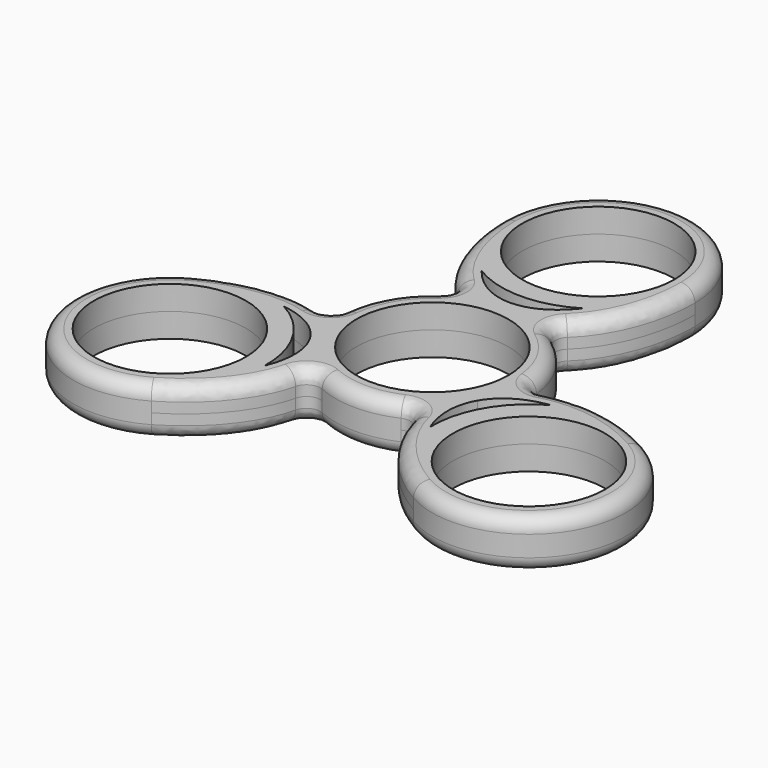
from build123d import *

# Parameters (mm, degrees)
F0_R     = 11
F1_DEPTH = 3.5
F2_F1_R  = 2
F2_F2_R  = 2


with BuildPart() as f1:
    # F0 (on Top) → F1 (new body, symmetric)
    with BuildSketch(Plane.XY):
        with BuildLine():
            add(Edge.make_bspline(
                [(-14, 30), (-14, 17.8068938204), (-5.8323690663, 12.7272727273)],
                knots=[1.5707963268, 1.5707963268, 1.5707963268, 2.7118929874, 2.7118929874, 2.7118929874], degree=2, weights=[1, 0.841604952, 1]))
            ThreePointArc((-5.8323690663, 12.7272727273), (-12.124355653, 7), (-13.9383260359, -1.312656588))
            ThreePointArc((-13.9383260359, -1.312656588), (-13.9167685556, -1.5243204946), (-13.8919969881, -1.7356323585))
            ThreePointArc((-13.8919969881, -1.7356323585), (-13.2718138334, -4.4563390324), (-12.1243556028, -7.0000000869))
            ThreePointArc((-12.1243556028, -7.0000000869), (-10.4952096602, -9.265558493), (-8.4491002081, -11.1630061217))
            ThreePointArc((-8.4491002081, -11.1630061217), (-8.2784845497, -11.2901148604), (-8.1059569696, -11.4146161393))
            ThreePointArc((-8.1059569696, -11.4146161393), (0, -14), (8.1059569696, -11.4146161393))
            ThreePointArc((8.1059569696, -11.4146161393), (8.2784845497, -11.2901148604), (8.4491002081, -11.1630061217))
            ThreePointArc((8.4491002081, -11.1630061217), (10.4952095782, -9.2655585859), (12.1243554789, -7.0000003015))
            ThreePointArc((12.1243554789, -7.0000003015), (13.271813794, -4.4563391499), (13.8919969881, -1.7356323585))
            ThreePointArc((13.8919969881, -1.7356323585), (13.9167685556, -1.5243204946), (13.9383260359, -1.312656588))
            ThreePointArc((13.9383260359, -1.312656588), (12.124355653, 7), (5.8323690663, 12.7272727273))
            add(Edge.make_bspline(
                [(5.8323690663, 12.7272727273), (14, 17.8068938204), (14, 30)],
                knots=[3.5712923197, 3.5712923197, 3.5712923197, 4.7123889804, 4.7123889804, 4.7123889804], degree=2, weights=[1, 0.841604952, 1]))
            ThreePointArc((14, 30), (0, 44), (-14, 30))
        make_face()
        Circle(F0_R, mode=Mode.SUBTRACT)
        with BuildLine():
            add(Edge.make_bspline(
                [(-7.3333333333, 18.07430412), (0, 8.533747416), (7.3333333333, 18.07430412)],
                knots=[2.4118649974, 2.4118649974, 2.4118649974, 3.8713203098, 3.8713203098, 3.8713203098], degree=2, weights=[1, 0.7453559925, 1]))
            ThreePointArc((-7.3333333333, 18.07430412), (0, 16), (7.3333333333, 18.07430412))
        make_face(mode=Mode.SUBTRACT)
        with Locations((0, 30)):
            Circle(F0_R, mode=Mode.SUBTRACT)
        with BuildLine():
            ThreePointArc((-13.8919969881, -1.7356323585), (-13.9167685556, -1.5243204946), (-13.9383260359, -1.312656588))
            add(Edge.make_bspline(
                [(-13.9383260359, -1.312656588), (-22.421222411, 3.2209087428), (-32.9807621135, -2.875644347)],
                knots=[3.5712923197, 3.5712923197, 3.5712923197, 4.7123889804, 4.7123889804, 4.7123889804], degree=2, weights=[1, 0.841604952, 1]))
            ThreePointArc((-32.9807621135, -2.875644347), (-38.1051177665, -22), (-18.9807621135, -27.124355653))
            add(Edge.make_bspline(
                [(-18.9807621135, -27.124355653), (-8.421222411, -21.0278025632), (-8.1059569696, -11.4146161393)],
                knots=[1.5707963268, 1.5707963268, 1.5707963268, 2.7118929874, 2.7118929874, 2.7118929874], degree=2, weights=[1, 0.841604952, 1]))
            ThreePointArc((-8.1059569696, -11.4146161393), (-8.2784845497, -11.2901148604), (-8.4491002081, -11.1630061217))
            ThreePointArc((-8.4491002081, -11.1630061217), (-10.4952096602, -9.265558493), (-12.1243556028, -7.0000000869))
            ThreePointArc((-12.1243556028, -7.0000000869), (-13.2718138334, -4.4563390324), (-13.8919969881, -1.7356323585))
        make_face()
        with Locations((-25.9807621135, -15)):
            Circle(F0_R, mode=Mode.SUBTRACT)
        with BuildLine():
            add(Edge.make_bspline(
                [(-12.1243556028, -7.0000000869), (-14.2251686452, -3.3612850489), (-19.3194731903, -2.6862990989)],
                knots=[3.1415926445, 3.1415926445, 3.1415926445, 3.8713203098, 3.8713203098, 3.8713203098], degree=2, weights=[1, 0.9341723573, 1]))
            add(Edge.make_bspline(
                [(-11.986139857, -15.3880050211), (-10.0235426179, -10.6387150253), (-12.1243556028, -7.0000000869)],
                knots=[2.4118649974, 2.4118649974, 2.4118649974, 3.1415926445, 3.1415926445, 3.1415926445], degree=2, weights=[1, 0.9341723606, 1]))
            ThreePointArc((-11.986139857, -15.3880050211), (-13.8564064606, -8), (-19.3194731903, -2.6862990989))
        make_face(mode=Mode.SUBTRACT)
        with BuildLine():
            add(Edge.make_bspline(
                [(32.9807621135, -2.875644347), (22.421222411, 3.2209087428), (13.9383260359, -1.312656588)],
                knots=[1.5707963268, 1.5707963268, 1.5707963268, 2.7118929874, 2.7118929874, 2.7118929874], degree=2, weights=[1, 0.841604952, 1]))
            ThreePointArc((13.9383260359, -1.312656588), (13.9167685556, -1.5243204946), (13.8919969881, -1.7356323585))
            ThreePointArc((13.8919969881, -1.7356323585), (13.271813794, -4.4563391499), (12.1243554789, -7.0000003015))
            ThreePointArc((12.1243554789, -7.0000003015), (10.4952095782, -9.2655585859), (8.4491002081, -11.1630061217))
            ThreePointArc((8.4491002081, -11.1630061217), (8.2784845497, -11.2901148604), (8.1059569696, -11.4146161393))
            add(Edge.make_bspline(
                [(8.1059569696, -11.4146161393), (8.421222411, -21.0278025632), (18.9807621135, -27.124355653)],
                knots=[3.5712923197, 3.5712923197, 3.5712923197, 4.7123889804, 4.7123889804, 4.7123889804], degree=2, weights=[1, 0.841604952, 1]))
            ThreePointArc((18.9807621135, -27.124355653), (38.1051177665, -22), (32.9807621135, -2.875644347))
        make_face()
        with Locations((25.9807621135, -15)):
            Circle(F0_R, mode=Mode.SUBTRACT)
        with BuildLine():
            add(Edge.make_bspline(
                [(12.1243554789, -7.0000003015), (10.0235426843, -10.6387151858), (11.986139857, -15.3880050211)],
                knots=[3.1415926852, 3.1415926852, 3.1415926852, 3.8713203098, 3.8713203098, 3.8713203098], degree=2, weights=[1, 0.9341723646, 1]))
            add(Edge.make_bspline(
                [(19.3194731903, -2.6862990989), (14.225168473, -3.3612850717), (12.1243554789, -7.0000003015)],
                knots=[2.4118649974, 2.4118649974, 2.4118649974, 3.1415926852, 3.1415926852, 3.1415926852], degree=2, weights=[1, 0.9341723533, 1]))
            ThreePointArc((19.3194731903, -2.6862990989), (13.8564064606, -8), (11.986139857, -15.3880050211))
        make_face(mode=Mode.SUBTRACT)
    extrude(amount=F1_DEPTH, both=True)

    # F2: fillet of radius 2 on 40 edges, made by hand

    # F2_f1
    f2_f1_edges = [f1.edges().sort_by_distance(p)[0] for p in [
        (-5.8323690663, 12.7272727273, -1.75),
        (-8.1059569696, -11.4146161393, -1.75),
        (-13.9383260359, -1.312656588, -1.75),
        (-13.9383260359, -1.312656588, 1.75),
        (-5.8323690663, 12.7272727273, 1.75),
        (8.1059569696, -11.4146161393, -1.75),
        (13.9383260359, -1.312656588, -1.75),
        (5.8323690663, 12.7272727273, -1.75),
        (5.8323690663, 12.7272727273, 1.75),
        (13.9383260359, -1.312656588, 1.75),
        (8.1059569696, -11.4146161393, 1.75),
        (-8.1059569696, -11.4146161393, 1.75),
    ]]
    fillet(f2_f1_edges, radius=F2_F1_R)

    # F2_f2
    f2_f2_edges = [f1.edges().sort_by_distance(p)[0] for p in [
        (-12.446293522, 21.3005366984, -3.5),
        (0, 44, -3.5),
        (0, 44, 3.5),
        (-38.1051177665, -22, -3.5),
        (-38.1051177665, -22, 3.5),
        (-12.223659134, -21.4290747222, -3.5),
        (-12.124355653, 7, -3.5),
        (-12.124355653, 7, 3.5),
        (-24.6699526561, 0.1285380239, -3.5),
        (12.223659134, -21.4290747222, -3.5),
        (38.1051177665, -22, -3.5),
        (38.1051177665, -22, 3.5),
        (12.124355653, 7, -3.5),
        (12.124355653, 7, 3.5),
        (12.223659134, -21.4290747222, 3.5),
        (24.6699526561, 0.1285380239, 3.5),
        (24.6699526561, 0.1285380239, -3.5),
        (-24.6699526561, 0.1285380239, 3.5),
        (-12.223659134, -21.4290747222, 3.5),
        (12.446293522, 21.3005366984, 3.5),
        (-12.446293522, 21.3005366984, 3.5),
        (12.446293522, 21.3005366984, -3.5),
        (7.385566687, 12.8300381313, -3.5),
        (-7.3855666873, 12.8300381307, 3.5),
        (7.385566687, 12.8300381313, 3.5),
        (-7.4183556091, -12.8111074378, 3.5),
        (-14.8039222962, -0.018930693, 3.5),
        (14.8039222968, -0.0189306934, -3.5),
        (14.8039222968, -0.0189306934, 3.5),
        (7.4183556097, -12.8111074381, 3.5),
        (7.4183556097, -12.8111074381, -3.5),
        (-14.8039222969, -0.0189306932, -3.5),
        (-7.385566687, 12.8300381313, -3.5),
        (-7.4183556091, -12.8111074378, -3.5),
    ]]
    fillet(f2_f2_edges, radius=F2_F2_R)


solid = f1.part
